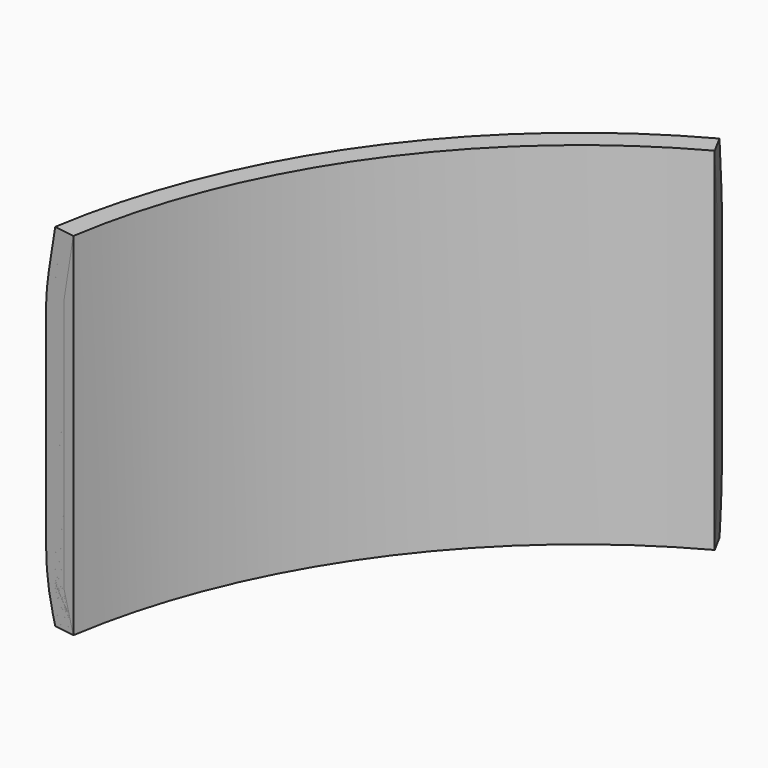
from build123d import *

# Parameters (mm, degrees)
F2_DEPTH = 33.6
F5_R     = 20


with BuildPart() as f2:
    # F1 (on Top) → F2 (new body)
    with BuildSketch(Plane.XY):
        with BuildLine():
            Line((0.9486013825, -1.7607258211), (0, 0))
            ThreePointArc((0, 0), (-19.8421488285, -17.5662997323), (-29.80036094, -42.1247965911))
            Line((-29.80036094, -42.1247965911), (-27.8242650699, -42.4330904643))
            ThreePointArc((-27.8242650699, -42.4330904643), (-18.2094047746, -18.721352482), (0.9486013825, -1.7607258211))
        make_face()
    extrude(amount=F2_DEPTH)


with BuildPart() as f4:
    # F4: sweep along a path in F4_path
    with BuildLine(Plane(origin=(0, 0, 33.6), x_dir=(0, -1, 0), z_dir=(0, 0, -1))) as f4_path:
        ThreePointArc((0, 0), (17.5662997323, 19.8421488285), (42.1247965911, 29.80036094))
    # F3 (on face) → F4 (sweep)
    with BuildSketch(Plane(origin=(-7.1238933736, -45.6625885183, 0), x_dir=(0.988047935, -0.1541469366, 0), z_dir=(-0.1541469366, -0.988047935, 0))):
        Polygon((-20.9507767409, 33.6), (-22.9507767409, 33.6), (-22.9507767409, 0), (-20.9507767409, 0), (-22.0040890729, 3.5874471068), (-22.0040890729, 27.6784074476), align=None)
        Polygon((-22.9507767409, 0), (-22.9507767409, 33.6), (-23.9604524097, 27.9237274081), (-23.9604524097, 3.5874471068), align=None)
    sweep(path=f4_path.line)

    # F5
    f5_edges = [f4.edges().sort_by_distance(p)[0] for p in [
        (-20.66642, -16.983185, 27.923727),
        (-20.66642, -16.983185, 3.587447),
    ]]
    fillet(f5_edges, radius=F5_R)


solid = Compound([f2.part, f4.part])
